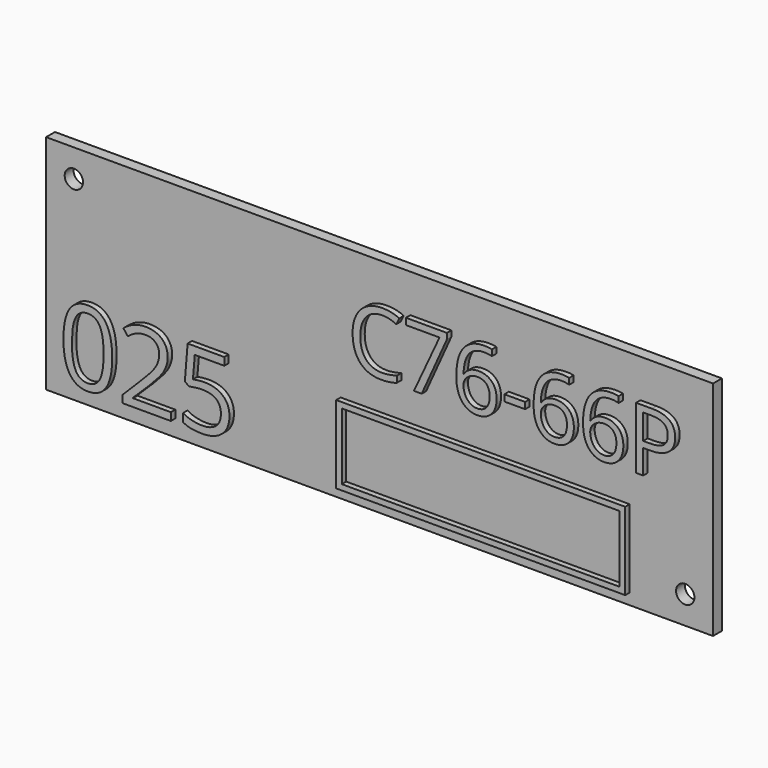
from build123d import *

# Parameters (mm, degrees)
F0_W         = 120
F0_H         = 40
F1_DEPTH     = 2
F3_D         = 3.3
F4_TEXT_SIZE = 15.5635715154
F5_DEPTH     = 1
F6_TEXT_SIZE = 18.5776487663
F7_DEPTH     = 1
F8_W         = 52
F8_H         = 14
F8_W_2       = 49.99999962
F8_H_2       = 11.99999962
F9_DEPTH     = 1


# Not quite as in the source:
# - Text() gives the source's letters only with a copy of the font that has no kerning and outlines rounded to 1/6400 em; it was checked with that copy


with BuildPart() as f1:
    # F0 (on Front) → F1 (new body)
    with BuildSketch(Plane.XZ):
        Rectangle(F0_W, F0_H)
    extrude(amount=F1_DEPTH)

    # F3 (through all)
    with Locations(Plane.XZ.offset(2)):
        with Locations((-55, 15), (55, -15)):
            Hole(F3_D / 2)

    # F4 (on face) → F5 (join)
    with BuildSketch(Plane.XZ.offset(2)):
        with Locations((-5, 2)):
            Text('C76-66P', F4_TEXT_SIZE, font='Open Sans', text_align=(TextAlign.LEFT, TextAlign.BOTTOM))
    extrude(amount=F5_DEPTH)

    # F6 (on face) → F7 (join)
    with BuildSketch(Plane.XZ.offset(2)):
        with Locations((-57, -17)):
            Text('025', F6_TEXT_SIZE, font='Open Sans', text_align=(TextAlign.LEFT, TextAlign.BOTTOM))
    extrude(amount=F7_DEPTH)

    # F8 (on face) → F9 (join)
    with BuildSketch(Plane.XZ.offset(2)):
        with Locations((19, -11)):
            Rectangle(F8_W, F8_H)
        with Locations((19, -11)):
            Rectangle(F8_W_2, F8_H_2, mode=Mode.SUBTRACT)
    extrude(amount=F9_DEPTH)


solid = f1.part
